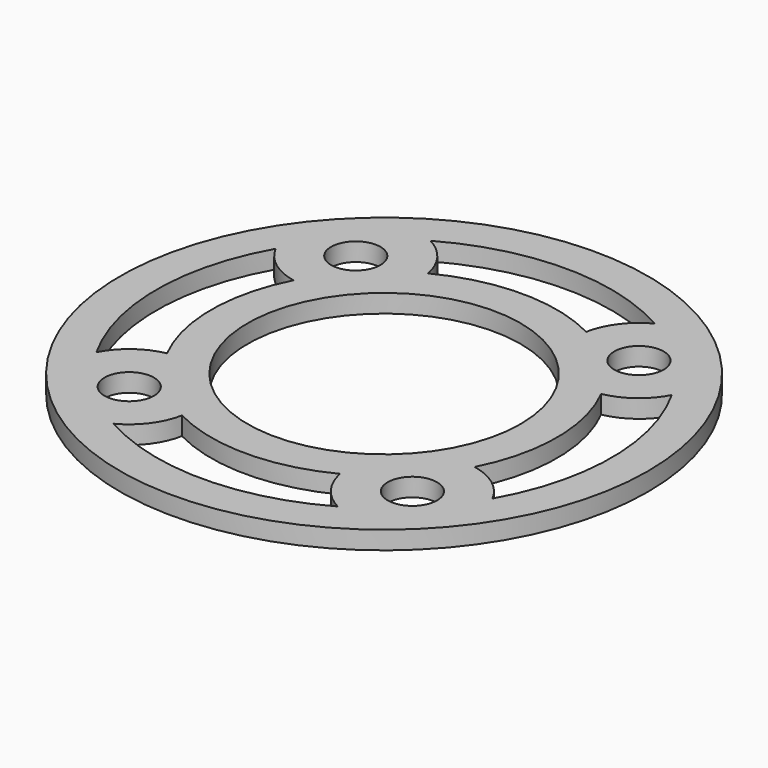
from build123d import *

# Parameters (mm, degrees)
F0_R            = 23.01875
F0_R_2          = 2.15265
F0_R_3          = 11.90625
F1_DEPTH        = 1.5875
F3_DEPTH        = 1.5875
F3_COPIES_COUNT = 4


# Not quite as in the source:
# - a pattern or mirror of a feature is missing from the dataset's text; its kind, count and spacing are read off the source's solid


with BuildPart() as f1:
    # F0 (on Top) → F1 (new body)
    with BuildSketch(Plane.XY):
        Circle(F0_R)
        with Locations((-12.3478521665, -12.3478521665)):
            Circle(F0_R_2, mode=Mode.SUBTRACT)
        with Locations((12.3478521665, -12.3478521665)):
            Circle(F0_R_2, mode=Mode.SUBTRACT)
        with Locations((-12.3478521665, 12.3478521665)):
            Circle(F0_R_2, mode=Mode.SUBTRACT)
        Circle(F0_R_3, mode=Mode.SUBTRACT)
        with Locations((12.3478521665, 12.3478521665)):
            Circle(F0_R_2, mode=Mode.SUBTRACT)
    extrude(amount=F1_DEPTH)

    # F2 (on face) → F3 (cut, through all)
    with BuildSketch(Plane.XY.offset(1.5875)):
        with BuildLine():
            ThreePointArc((-9.7719120136, 17.2709047146), (-7.8938999882, 15.6696324205), (-6.8946489019, 13.4129757356))
            ThreePointArc((-6.8946489019, 13.4129757356), (0, 15.08125), (6.8946489019, 13.4129757356))
            ThreePointArc((6.8946489019, 13.4129757356), (7.8938999882, 15.6696324205), (9.7719120136, 17.2709047146))
            ThreePointArc((9.7719120136, 17.2709047146), (0, 19.84375), (-9.7719120136, 17.2709047146))
        make_face()
    f3 = extrude(amount=-F3_DEPTH, mode=Mode.SUBTRACT)

    # F3_copies: F3 ×4 about axis
    f3_copies_axis = Axis((0, 0, 0), (0, 0, 1))
    for i in range(1, F3_COPIES_COUNT):
        add(f3.rotate(f3_copies_axis, i * 360 / F3_COPIES_COUNT), mode=Mode.SUBTRACT)


solid = f1.part
